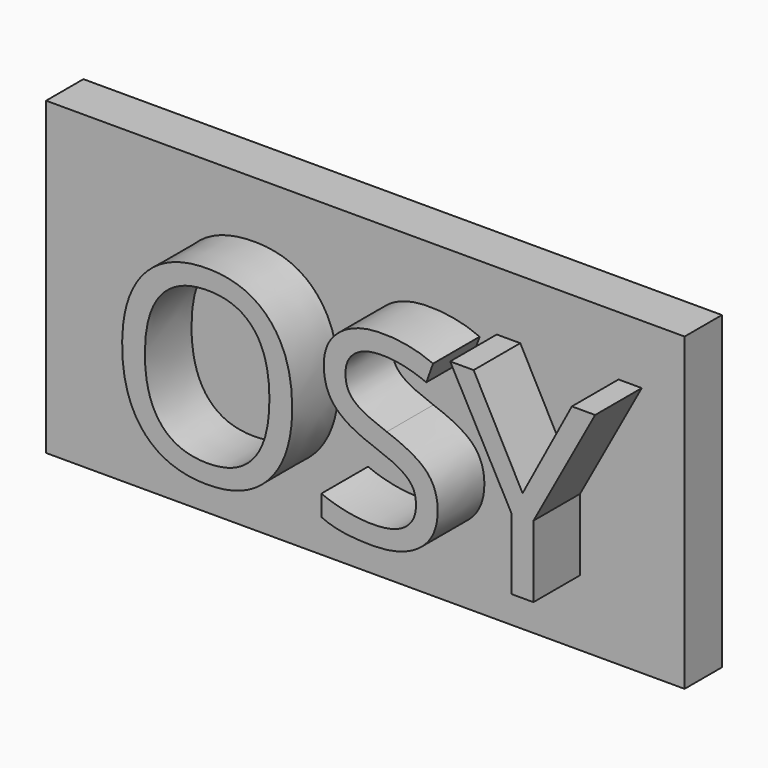
from build123d import *

# Parameters (mm, degrees)
F0_W         = 69.5349276066
F0_H         = 33.7761230767
F1_DEPTH     = 5.08
F2_TEXT_SIZE = 28.2002289573
F3_DEPTH     = 6.35


# Not quite as in the source:
# - Text() gives the source's letters only with a copy of the font that has no kerning and outlines rounded to 1/6400 em; it was checked with that copy


with BuildPart() as f1:
    # F0 (on Front) → F1 (new body)
    with BuildSketch(Plane.XZ):
        with Locations((34.7674638033, 16.8880615383)):
            Rectangle(F0_W, F0_H)
    extrude(amount=F1_DEPTH)

    # F2 (on face) → F3 (join)
    with BuildSketch(Plane.XZ.offset(5.08)):
        with Locations((11.6392467171, 7.1894442663)):
            Text('OSY', F2_TEXT_SIZE, font='Open Sans', text_align=(TextAlign.LEFT, TextAlign.BOTTOM))
    extrude(amount=F3_DEPTH)


solid = f1.part
